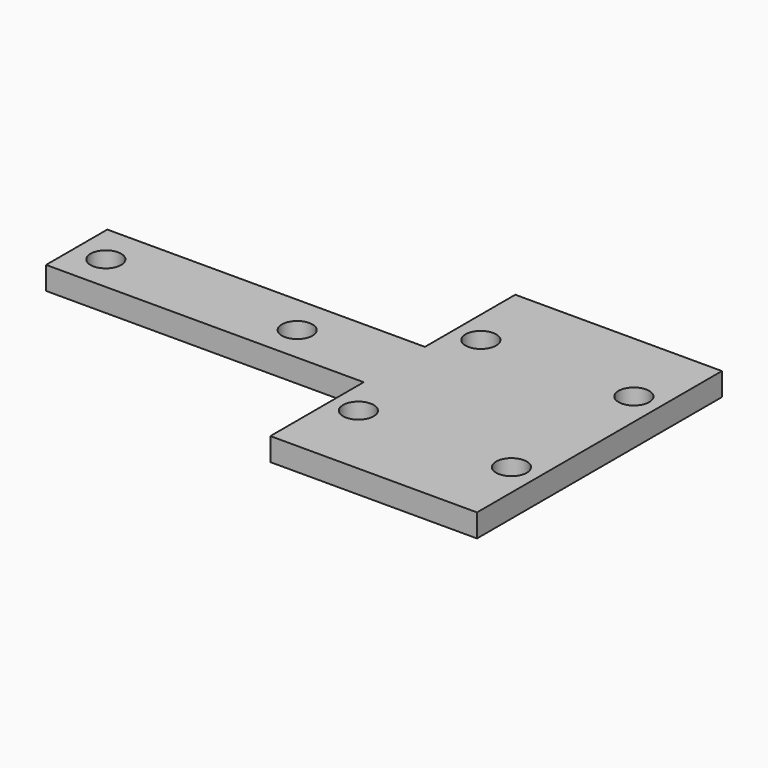
from build123d import *

# Parameters (mm, degrees)
F1_DEPTH = 3
F2_D     = 4


with BuildPart() as f1:
    # F0 (on Top) → F1 (new body)
    with BuildSketch(Plane.XY):
        Polygon((-13.5, -20), (13.5, -20), (13.5, 20), (-13.5, 20), (-13.5, 5.2414399013), (-55, 5.2414399013), (-55, -4.7585600987), (-13.5, -4.7585600987), align=None)
    extrude(amount=F1_DEPTH)

    # F2 (through all)
    with Locations(Plane(origin=(0, 0, 0), x_dir=(1, 0, 0), z_dir=(0, 0, -1))):
        with Locations((-51, 0), (-26, 0), (-10, 10), (10, -10), (10, 10), (-10, -10)):
            Hole(F2_D / 2)


solid = f1.part
